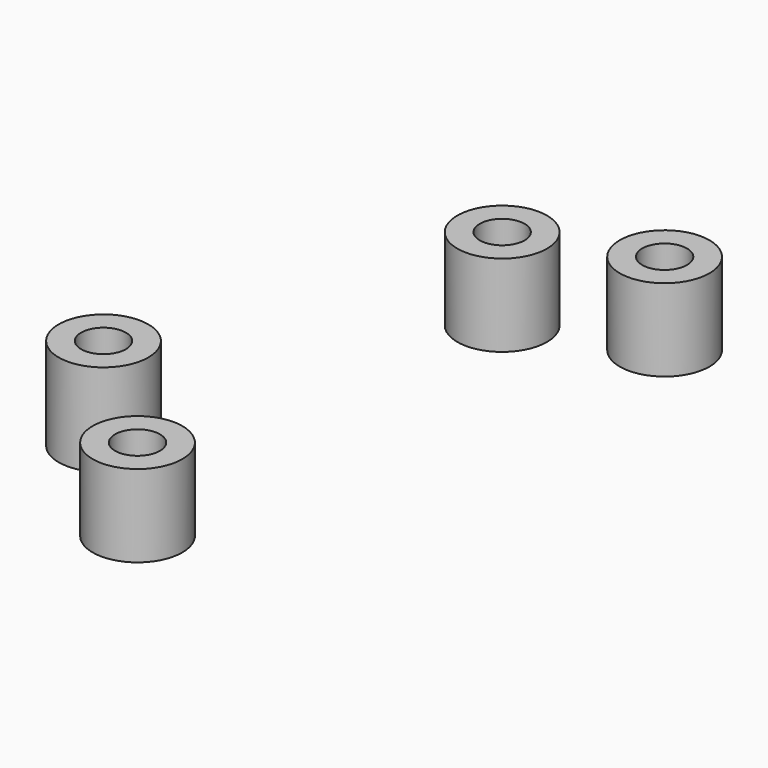
from build123d import *

# Parameters (mm, degrees)
F0_R     = 12
F0_R_2   = 6
F1_DEPTH = 22
F2_DEPTH = 24.7


# Not quite as in the source:
# - a feature names something its author has since deleted; it is built from what else it names


with BuildPart() as f1:
    # F0 (on Top) → F1 (new body)
    with BuildSketch(Plane.XY):
        with Locations((-34.3365694268, 61)):
            Circle(F0_R)
        with Locations((-34.3365694268, 61)):
            Circle(F0_R_2, mode=Mode.SUBTRACT)
    extrude(amount=F1_DEPTH)


with BuildPart() as f1b:
    # F0 (on Top) → F1, piece 2 (new body)
    with BuildSketch(Plane.XY):
        with Locations((-34.3365694268, -61)):
            Circle(F0_R)
        with Locations((-34.3365694268, -61)):
            Circle(F0_R_2, mode=Mode.SUBTRACT)
    extrude(amount=F1_DEPTH)


with BuildPart() as f1c:
    # F0 (on Top) → F1, piece 3 (new body)
    with BuildSketch(Plane.XY):
        with Locations((-0.860383961, 73.4949640414)):
            Circle(F0_R)
        with Locations((-0.860383961, 73.4949640414)):
            Circle(F0_R_2, mode=Mode.SUBTRACT)
    extrude(amount=F1_DEPTH)


with BuildPart() as f2:
    # F0 (on Top) → F2 (new body)
    with BuildSketch(Plane.XY):
        with Locations((-65.3908093134, -33.5602749889)):
            Circle(F0_R)
        with Locations((-65.3908093134, -33.5602749889)):
            Circle(F0_R_2, mode=Mode.SUBTRACT)
    extrude(amount=F2_DEPTH)


solid = Compound([f1.part, f1b.part, f1c.part, f2.part])
